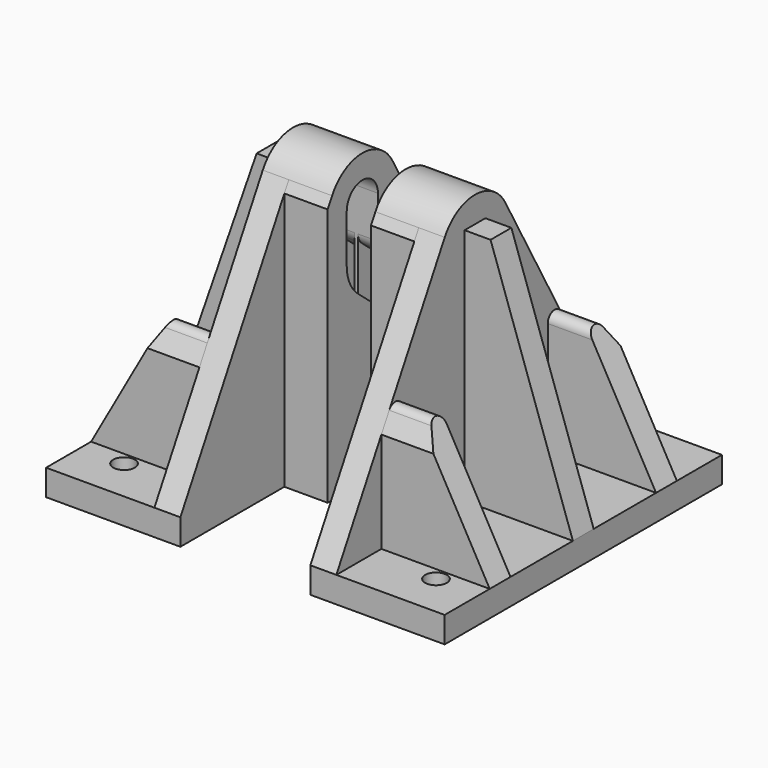
from build123d import *

# Parameters (mm, degrees)
F1_DEPTH       = 6
F3_DEPTH       = 61
F5_DEPTH       = 25
F6_W           = 25
F6_H           = 6
F7_DEPTH       = 55
F9_DEPTH       = 66
F11_DEPTH      = 10
F13_DEPTH      = 10
F14_R          = 2
F17_DEPTH      = 0.4
F17_DEPTH_BACK = 0.4
F19_DEPTH      = 0.8
F20_R          = 2.5
F21_DEPTH      = 20
F22_R          = 2
F24_DEPTH      = 14.1
F26_DEPTH      = 9.9
F28_DEPTH      = 6.1
F29_T1_DEPTH   = 25.1731750977


# Not quite as in the source:
# - a fillet or chamfer that OpenCascade refuses, or shapes differently, is made with other operations: its cross-section is extruded or revolved along the edge and cut away or added


with BuildPart() as f1:
    # F0 (on Top) → F1 (new body)
    with BuildSketch(Plane.XY):
        Polygon((15.5, 40), (-15.5, 40), (-15.5, -40), (15.5, -40), (15.5, -10), (25.5, -10), (25.5, 16), (15.5, 16), align=None)
    extrude(amount=F1_DEPTH)

    # F2 (on face) → F3 (join)
    with BuildSketch(Plane.XY.offset(6)):
        Polygon((15.5, 16), (15.5, 40), (9.5, 40), (9.5, -40), (15.5, -40), (15.5, -10), align=None)
    extrude(amount=F3_DEPTH)

    # F4 (on face) → F5 (cut)
    with BuildSketch(Plane(origin=(9.5, 0, 0), x_dir=(0, -1, 0), z_dir=(-1, 0, 0))):
        with BuildLine():
            ThreePointArc((-8.7264736489, 61.8835087442), (0, 67), (8.7264736489, 61.8835087442))
            Line((8.7264736489, 61.8835087442), (40, 6))
            Line((40, 6), (42.4536168575, 71.3308081031))
            Line((42.4536168575, 71.3308081031), (-55.2879087627, 71.3308081031))
            Line((-55.2879087627, 71.3308081031), (-55.2879087627, 6))
            Line((-55.2879087627, 6), (-40, 6))
            Line((-40, 6), (-8.7264736489, 61.8835087442))
        make_face()
    extrude(amount=-F5_DEPTH, mode=Mode.SUBTRACT)

    # F6 (on face) → F7 (join)
    with BuildSketch(Plane.XY.offset(6)):
        with Locations((-3, 0)):
            Rectangle(F6_W, F6_H)
        with Locations((-3, -24)):
            Rectangle(F6_W, F6_H)
        with Locations((-3, 24)):
            Rectangle(F6_W, F6_H)
    extrude(amount=F7_DEPTH)

    # F8 (on face) → F9 (cut)
    with BuildSketch(Plane.YZ.offset(9.5)):
        with BuildLine():
            Line((-71.4004188776, 87.6169577241), (-40, 6))
            Line((-40, 6), (-27, 29.2300510508))
            Line((-27, 29.2300510508), (-21, 39.9516130743))
            Line((-21, 39.9516130743), (-8.7264736489, 61.8835087442))
            ThreePointArc((-8.7264736489, 61.8835087442), (-6.3084751181, 64.7590683516), (-3, 66.5393920142))
            ThreePointArc((-3, 66.5393920142), (0, 67), (3, 66.5393920142))
            ThreePointArc((3, 66.5393920142), (6.3084751181, 64.7590683516), (8.7264736489, 61.8835087442))
            Line((8.7264736489, 61.8835087442), (21, 39.9516130743))
            Line((21, 39.9516130743), (27, 29.2300510508))
            Line((27, 29.2300510508), (40, 6))
            Line((40, 6), (67.9079666734, 87.6169577241))
            Line((67.9079666734, 87.6169577241), (-71.4004188776, 87.6169577241))
        make_face()
    extrude(amount=-F9_DEPTH, mode=Mode.SUBTRACT)

    # F10 (on face) → F11 (join, through all)
    with BuildSketch(Plane.YZ.offset(15.5)):
        with BuildLine():
            Line((-10, 59.6078101173), (-10, 6))
            Line((-10, 6), (16, 6))
            Line((16, 6), (16, 48.8862480938))
            Line((16, 48.8862480938), (8.7264736489, 61.8835087442))
            ThreePointArc((8.7264736489, 61.8835087442), (0, 67), (-8.7264736489, 61.8835087442))
            Line((-8.7264736489, 61.8835087442), (-10, 59.6078101173))
        make_face()
    extrude(amount=F11_DEPTH)

    # F12 (on face) → F13 (cut, through all)
    with BuildSketch(Plane.YZ.offset(25.5)):
        with BuildLine():
            ThreePointArc((0, 61.5), (-3.1819805153, 60.1819805153), (-4.5, 57))
            Line((-4.5, 57), (-4.5, 45.8414354094))
            ThreePointArc((-4.5, 45.8414354094), (-3.6567700833, 42.0378710538), (-1.2850884872, 38.9470354214))
            Line((-1.2850884872, 38.9470354214), (16, 24.4431240469))
            Line((16, 24.4431240469), (16, 36.1917896509))
            Line((16, 36.1917896509), (5.5716371709, 44.9422250545))
            ThreePointArc((5.5716371709, 44.9422250545), (4.7810766389, 45.9725035987), (4.5, 47.2403583839))
            Line((4.5, 47.2403583839), (4.5, 57))
            ThreePointArc((4.5, 57), (3.1819805153, 60.1819805153), (0, 61.5))
        make_face()
    extrude(amount=-F13_DEPTH, mode=Mode.SUBTRACT)

    # F14
    f14_edges = [f1.edges().sort_by_distance(p)[0] for p in [
        (20.5, 16, 36.19179),
        (20.5, 16, 24.443124),
    ]]
    fillet(f14_edges, radius=F14_R)

    # F16 (on offset) → F17 (join, two sides)
    with BuildSketch(Plane.YZ.offset(20.5)) as f17_sk:
        Polygon((16, 40.4808034919), (4.5, 50.1304492505), (4.5, 33.1601544891), (16, 23.5105087306), align=None)
    extrude(amount=F17_DEPTH)
    extrude(f17_sk.sketch, amount=-F17_DEPTH_BACK)

    # F18 (on face) → F19 (join)
    with BuildSketch(Plane.YZ.offset(25.5)):
        with BuildLine():
            ThreePointArc((16, 40.4808034919), (14.8452365235, 38.6681879179), (12.7144247806, 38.9487146057))
            Line((12.7144247806, 38.9487146057), (5.5716371709, 44.9422250545))
            ThreePointArc((5.5716371709, 44.9422250545), (4.7810766389, 45.9725035987), (4.5, 47.2403583839))
            Line((4.5, 47.2403583839), (4.5, 34.0927698054))
            Line((4.5, 34.0927698054), (15.2855752194, 25.0425976168))
            ThreePointArc((15.2855752194, 25.0425976168), (15.8126155741, 24.3557452541), (16, 23.5105087306))
            Line((16, 23.5105087306), (16, 40.4808034919))
        make_face()
    extrude(amount=-F19_DEPTH)

    # F20 (on face) → F21 (cut)
    with BuildSketch(Plane(origin=(0, 0, 0), x_dir=(1, 0, 0), z_dir=(0, 0, -1))):
        with Locations((-5.5, 0)):
            Circle(F20_R)
        with Locations((-5.5, 30)):
            Circle(F20_R)
        with Locations((-5.5, -30)):
            Circle(F20_R)
    extrude(amount=-F21_DEPTH, mode=Mode.SUBTRACT)

    # F22
    f22_edges = [f1.edges().sort_by_distance(p)[0] for p in [
        (-8, 0, 20),
    ]]
    fillet(f22_edges, radius=F22_R)

    # F23 (on face) → F24 (cut)
    with BuildSketch(Plane.XZ.offset(27)):
        Polygon((3.5, 39.9516130743), (9.5, 39.9516130743), (9.5, 46.4005209506), (-37.9068218172, 46.4005209506), (-37.9068218172, 6), (-15.5, 6), align=None)
    extrude(amount=-F24_DEPTH, mode=Mode.SUBTRACT)

    # F25 (on face) → F26 (cut)
    with BuildSketch(Plane(origin=(0, 27, 0), x_dir=(-1, 0, 0), z_dir=(0, 1, 0))):
        Polygon((-9.5, 49.5710298419), (-9.5, 39.9516130743), (-3.5, 39.9516130743), (15.5, 6), (21.0043340921, 6), (21.0043340921, 49.5710298419), align=None)
    extrude(amount=-F26_DEPTH, mode=Mode.SUBTRACT)

    # F27 (on face) → F28 (cut)
    with BuildSketch(Plane(origin=(0, 3, 0), x_dir=(-1, 0, 0), z_dir=(0, 1, 0))):
        Polygon((-9.5, 63.8725236058), (-9.5, 61), (-3.5, 61), (15.5, 6), (33.5027240217, 48.3329854906), (22.2862139344, 65.7419413328), align=None)
    extrude(amount=-F28_DEPTH, mode=Mode.SUBTRACT)

    # F29: fillet of radius 2 on 2 edges, made by hand

    # F29_s2 → F29_t1 (cut)
    with BuildSketch(Plane.YZ.offset(-15.6731750977)):
        with BuildLine():
            ThreePointArc((24.7452947298, 33.259044784), (22.4953166634, 34.2176194314), (21, 32.2823430352))
            Line((21, 32.2823430352), (21, 39.9516130743))
            Line((21, 39.9516130743), (24.7452947298, 33.259044784))
        make_face()
        with BuildLine():
            ThreePointArc((-21, 32.2823430352), (-22.4953166634, 34.2176194314), (-24.7452947298, 33.259044784))
            Line((-24.7452947298, 33.259044784), (-21, 39.9516130743))
            Line((-21, 39.9516130743), (-21, 32.2823430352))
        make_face()
    extrude(amount=F29_T1_DEPTH, mode=Mode.SUBTRACT)


with BuildPart() as f31_1:
    # F31: instance of F1
    add(f1.part.mirror(Plane(origin=(30.5, 2.9102814818, 28.9120815195), x_dir=(0, 1, 0), z_dir=(1, 0, 0))))


solid = Compound([f1.part, f31_1.part])
